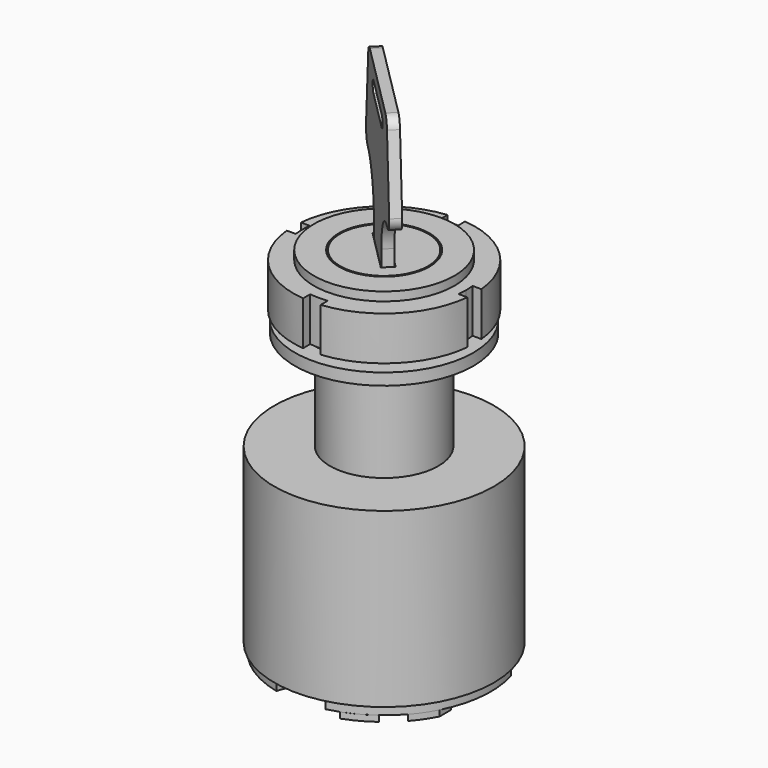
from build123d import *

# Parameters (mm, degrees)
F3_R      = 12
F4_DEPTH  = 7.5
F6_DEPTH  = 0.5
F7_R      = 7.75
F7_R_2    = 7.5
F8_DEPTH  = 0.5
F11_DEPTH = 0.875
F13_DEPTH = 1.5
F16_DEPTH = 1
F17_DEPTH = 1
F18_DEPTH = 1


# Not quite as in the source:
# - a feature names something its author has since deleted; it is built from what else it names


with BuildPart() as f1:
    # F0 (on Front) → F1 (revolve)
    with BuildSketch(Plane.XZ):
        Polygon((0, 59), (0, 0), (18.75, 0), (18.75, 29.5), (9.25, 29.5), (9.25, 44.5), (15.25, 46.5), (15.25, 48.5), (12, 48.5), (12, 59), align=None)
    revolve(axis=Axis((0, 0, 29.5), (0, 0, -1)))

    # F5 (on face) → F6 (cut)
    with BuildSketch(Plane.XY.offset(57.5)):
        with BuildLine():
            ThreePointArc((14.6735305908, 1.5), (14.7308702427, 0.7509739627), (14.75, 0))
            ThreePointArc((14.75, 0), (14.7308702427, -0.7509739627), (14.6735305908, -1.5))
            Line((14.6735305908, -1.5), (15.4272486205, -1.5))
            ThreePointArc((15.4272486205, -1.5), (15.4818014717, -0.750881609), (15.5, 0))
            ThreePointArc((15.5, 0), (15.4818014717, 0.750881609), (15.4272486205, 1.5))
            Line((15.4272486205, 1.5), (14.6735305908, 1.5))
        make_face()
        with BuildLine():
            ThreePointArc((-1.5, 14.6735305908), (0, 14.75), (1.5, 14.6735305908))
            Line((1.5, 14.6735305908), (1.5, 15.4272486205))
            ThreePointArc((1.5, 15.4272486205), (0, 15.5), (-1.5, 15.4272486205))
            Line((-1.5, 15.4272486205), (-1.5, 14.6735305908))
        make_face()
        with BuildLine():
            Line((1.5, -15.4272486205), (1.5, -14.6735305908))
            ThreePointArc((1.5, -14.6735305908), (0, -14.75), (-1.5, -14.6735305908))
            Line((-1.5, -14.6735305908), (-1.5, -15.4272486205))
            ThreePointArc((-1.5, -15.4272486205), (0, -15.5), (1.5, -15.4272486205))
        make_face()
        with BuildLine():
            ThreePointArc((-14.6735305908, -1.5), (-14.75, 0), (-14.6735305908, 1.5))
            Line((-14.6735305908, 1.5), (-15.4272486205, 1.5))
            ThreePointArc((-15.4272486205, 1.5), (-15.5, 0), (-15.4272486205, -1.5))
            Line((-15.4272486205, -1.5), (-14.6735305908, -1.5))
        make_face()
    extrude(amount=-F6_DEPTH, mode=Mode.SUBTRACT)

    # F7 (on face) → F8 (cut)
    with BuildSketch(Plane.XY.offset(59)):
        Circle(F7_R)
        Circle(F7_R_2, mode=Mode.SUBTRACT)
        Polygon((-2.8284271247, 4.2426406871), (-4.2426406871, 2.8284271247), (2.8284271247, -4.2426406871), (4.2426406871, -2.8284271247), (0, 1.4142135624), align=None)
    extrude(amount=-F8_DEPTH, mode=Mode.SUBTRACT)


with BuildPart() as f4:
    # F3 (on offset) → F4 (new body)
    with BuildSketch(Plane.XY.offset(50)):
        with BuildLine():
            Line((-1.5, 13.9194109071), (-1.5, 15.4272486205))
            ThreePointArc((-1.5, 15.4272486205), (-10.9601551084, 10.9601551084), (-15.4272486205, 1.5))
            Line((-15.4272486205, 1.5), (-13.9194109071, 1.5))
            ThreePointArc((-13.9194109071, 1.5), (-9.8994949366, 9.8994949366), (-1.5, 13.9194109071))
        make_face()
        with BuildLine():
            ThreePointArc((-1.5, -13.9194109071), (-9.8994949366, -9.8994949366), (-13.9194109071, -1.5))
            Line((-13.9194109071, -1.5), (-15.4272486205, -1.5))
            ThreePointArc((-15.4272486205, -1.5), (-10.9601551084, -10.9601551084), (-1.5, -15.4272486205))
            Line((-1.5, -15.4272486205), (-1.5, -13.9194109071))
        make_face()
        with BuildLine():
            ThreePointArc((13.9194109071, -1.5), (9.8994949366, -9.8994949366), (1.5, -13.9194109071))
            Line((1.5, -13.9194109071), (1.5, -15.4272486205))
            ThreePointArc((1.5, -15.4272486205), (10.9601551084, -10.9601551084), (15.4272486205, -1.5))
            Line((15.4272486205, -1.5), (13.9194109071, -1.5))
        make_face()
        with BuildLine():
            ThreePointArc((0, 14), (-0.7510816537, 13.979838209), (-1.5, 13.9194109071))
            ThreePointArc((-1.5, 13.9194109071), (-9.8994949366, 9.8994949366), (-13.9194109071, 1.5))
            ThreePointArc((-13.9194109071, 1.5), (-14, 0), (-13.9194109071, -1.5))
            ThreePointArc((-13.9194109071, -1.5), (-9.8994949366, -9.8994949366), (-1.5, -13.9194109071))
            ThreePointArc((-1.5, -13.9194109071), (0, -14), (1.5, -13.9194109071))
            ThreePointArc((1.5, -13.9194109071), (9.8994949366, -9.8994949366), (13.9194109071, -1.5))
            ThreePointArc((13.9194109071, -1.5), (13.979838209, -0.7510816537), (14, 0))
            ThreePointArc((14, 0), (13.979838209, 0.7510816537), (13.9194109071, 1.5))
            ThreePointArc((13.9194109071, 1.5), (9.8994949366, 9.8994949366), (1.5, 13.9194109071))
            ThreePointArc((1.5, 13.9194109071), (0.7510816537, 13.979838209), (0, 14))
        make_face()
        Circle(F3_R, mode=Mode.SUBTRACT)
        with BuildLine():
            Line((1.5, 15.4272486205), (1.5, 13.9194109071))
            ThreePointArc((1.5, 13.9194109071), (9.8994949366, 9.8994949366), (13.9194109071, 1.5))
            Line((13.9194109071, 1.5), (15.4272486205, 1.5))
            ThreePointArc((15.4272486205, 1.5), (10.9601551084, 10.9601551084), (1.5, 15.4272486205))
        make_face()
    extrude(amount=F4_DEPTH)


with BuildPart() as f11:
    # F10 (on offset) → F11 (new body, symmetric)
    with BuildSketch(Plane(origin=(0, 0, 0), x_dir=(0.7071067812, -0.7071067812, 0), z_dir=(-0.7071067812, -0.7071067812, 0))):
        with BuildLine():
            Line((-4.5, 58.5), (0, 58.5))
            Line((0, 58.5), (4.5, 58.5))
            Line((4.5, 58.5), (4.5, 61.5))
            ThreePointArc((4.5, 61.5), (6.5502525317, 66.4497474683), (11.5, 68.5))
            Line((11.5, 68.5), (12.0152075807, 68.5))
            ThreePointArc((12.0152075807, 68.5), (13.5732171306, 69.2459640187), (13.9690076155, 70.9273937576))
            Line((13.9690076155, 70.9273937576), (11.3440076155, 82.9273937576))
            ThreePointArc((11.3440076155, 82.9273937576), (10.644243562, 84.0580095499), (9.3902075807, 84.5))
            Line((9.3902075807, 84.5), (0, 84.5))
            Line((0, 84.5), (-9.3902075807, 84.5))
            ThreePointArc((-9.3902075807, 84.5), (-10.644243562, 84.0580095499), (-11.3440076155, 82.9273937576))
            Line((-11.3440076155, 82.9273937576), (-13.9690076155, 70.9273937576))
            ThreePointArc((-13.9690076155, 70.9273937576), (-13.5732171306, 69.2459640187), (-12.0152075807, 68.5))
            Line((-12.0152075807, 68.5), (-11.5, 68.5))
            ThreePointArc((-11.5, 68.5), (-6.5502525317, 66.4497474683), (-4.5, 61.5))
            Line((-4.5, 61.5), (-4.5, 58.5))
        make_face()
        with BuildLine():
            Line((-5, 82), (0, 82))
            Line((0, 82), (5, 82))
            ThreePointArc((5, 82), (6, 81), (5, 80))
            Line((5, 80), (0, 80))
            Line((0, 80), (-5, 80))
            ThreePointArc((-5, 80), (-6, 81), (-5, 82))
        make_face(mode=Mode.SUBTRACT)
    extrude(amount=F11_DEPTH, both=True)


with BuildPart() as f13:
    # F12 (on face) → F13 (new body)
    with BuildSketch(Plane(origin=(0, 0, 0), x_dir=(1, 0, 0), z_dir=(0, 0, -1))):
        with BuildLine():
            ThreePointArc((4.1808768461, 17.7646494139), (0, 14.2780423647), (-4.1808768461, 17.7646494139))
            ThreePointArc((-4.1808768461, 17.7646494139), (-15.8049636191, 9.125), (-17.4750761048, -5.2615791481))
            ThreePointArc((-17.4750761048, -5.2615791481), (-12.3651474041, -7.1390211823), (-13.2941992587, -12.5030702658))
            ThreePointArc((-13.2941992587, -12.5030702658), (0, -18.25), (13.2941992587, -12.5030702658))
            ThreePointArc((13.2941992587, -12.5030702658), (12.3651474041, -7.1390211823), (17.4750761048, -5.2615791481))
            ThreePointArc((17.4750761048, -5.2615791481), (15.8049636191, 9.125), (4.1808768461, 17.7646494139))
        make_face()
    extrude(amount=F13_DEPTH)

    # F15 (on face) → F18 (join)
    with BuildSketch(Plane(origin=(0, 0, -1.5), x_dir=(1, 0, 0), z_dir=(0, 0, -1))):
        with BuildLine():
            Line((16.1942188134, 6.1666581865), (16.1942188134, 8.4148545455))
            ThreePointArc((16.1942188134, 8.4148545455), (15.0551666883, 10.315253559), (13.6942188134, 12.0636176618))
            Line((13.6942188134, 12.0636176618), (13.6942188134, 8.6666581865))
            ThreePointArc((13.6942188134, 8.6666581865), (13.547772204, 8.3131047959), (13.1942188134, 8.1666581865))
            Line((13.1942188134, 8.1666581865), (6.6942188134, 8.1666581865))
            ThreePointArc((6.6942188134, 8.1666581865), (6.3406654228, 8.0202115771), (6.1942188134, 7.6666581865))
            Line((6.1942188134, 7.6666581865), (6.1942188134, 6.1666581865))
            ThreePointArc((6.1942188134, 6.1666581865), (6.3406654228, 5.8131047959), (6.6942188134, 5.6666581865))
            Line((6.6942188134, 5.6666581865), (15.6942188134, 5.6666581865))
            ThreePointArc((15.6942188134, 5.6666581865), (16.047772204, 5.8131047959), (16.1942188134, 6.1666581865))
        make_face()
    extrude(amount=F18_DEPTH)


with BuildPart() as f16:
    # F15 (on face) → F16 (new body)
    with BuildSketch(Plane(origin=(0, 0, -1.5), x_dir=(1, 0, 0), z_dir=(0, 0, -1))):
        with BuildLine():
            Line((-5, -16.25), (-5, -17.5517093185))
            ThreePointArc((-5, -17.5517093185), (0, -18.25), (5, -17.5517093185))
            Line((5, -17.5517093185), (5, -12.75))
            ThreePointArc((5, -12.75), (5.1464466094, -12.3964466094), (5.5, -12.25))
            Line((5.5, -12.25), (10.5, -12.25))
            ThreePointArc((10.5, -12.25), (10.8535533906, -12.1035533906), (11, -11.75))
            Line((11, -11.75), (11, -2.75))
            ThreePointArc((11, -2.75), (10.8535533906, -2.3964466094), (10.5, -2.25))
            Line((10.5, -2.25), (9, -2.25))
            ThreePointArc((9, -2.25), (8.6464466094, -2.3964466094), (8.5, -2.75))
            Line((8.5, -2.75), (8.5, -9.25))
            ThreePointArc((8.5, -9.25), (8.3535533906, -9.6035533906), (8, -9.75))
            Line((8, -9.75), (3, -9.75))
            ThreePointArc((3, -9.75), (2.6464466094, -9.6035533906), (2.5, -9.25))
            Line((2.5, -9.25), (2.5, -2.75))
            ThreePointArc((2.5, -2.75), (2.3535533906, -2.3964466094), (2, -2.25))
            Line((2, -2.25), (0.5, -2.25))
            ThreePointArc((0.5, -2.25), (0.1464466094, -2.3964466094), (0, -2.75))
            Line((0, -2.75), (0, -3.0306600966))
            Line((0, -3.0306600966), (-4.25, -3.0306600966))
            Line((-4.25, -3.0306600966), (-4.25, 5.5))
            ThreePointArc((-4.25, 5.5), (-4.3964466094, 5.8535533906), (-4.75, 6))
            Line((-4.75, 6), (-6.25, 6))
            ThreePointArc((-6.25, 6), (-6.6035533906, 5.8535533906), (-6.75, 5.5))
            Line((-6.75, 5.5), (-6.75, -1))
            ThreePointArc((-6.75, -1), (-6.8964466094, -1.3535533906), (-7.25, -1.5))
            Line((-7.25, -1.5), (-12.25, -1.5))
            ThreePointArc((-12.25, -1.5), (-12.6035533906, -1.3535533906), (-12.75, -1))
            Line((-12.75, -1), (-12.75, 5.5))
            ThreePointArc((-12.75, 5.5), (-12.8964466094, 5.8535533906), (-13.25, 6))
            Line((-13.25, 6), (-14.75, 6))
            ThreePointArc((-14.75, 6), (-15.1035533906, 5.8535533906), (-15.25, 5.5))
            Line((-15.25, 5.5), (-15.25, -3.5))
            ThreePointArc((-15.25, -3.5), (-15.1035533906, -3.8535533906), (-14.75, -4))
            Line((-14.75, -4), (-4.75, -4))
            ThreePointArc((-4.75, -4), (-4.3964466094, -3.8535533906), (-4.25, -3.5))
            Line((-4.25, -3.5), (-4.25, -3.1480044127))
            Line((-4.25, -3.1480044127), (0, -3.1480044127))
            Line((0, -3.1480044127), (0, -6.75))
            ThreePointArc((0, -6.75), (-0.1464466094, -7.1035533906), (-0.5, -7.25))
            Line((-0.5, -7.25), (-4.5, -7.25))
            ThreePointArc((-4.5, -7.25), (-4.8535533906, -7.3964466094), (-5, -7.75))
            Line((-5, -7.75), (-5, -9.25))
            ThreePointArc((-5, -9.25), (-4.8535533906, -9.6035533906), (-4.5, -9.75))
            Line((-4.5, -9.75), (2, -9.75))
            ThreePointArc((2, -9.75), (2.3535533906, -9.8964466094), (2.5, -10.25))
            Line((2.5, -10.25), (2.5, -15.25))
            ThreePointArc((2.5, -15.25), (2.3535533906, -15.6035533906), (2, -15.75))
            Line((2, -15.75), (0, -15.75))
            Line((0, -15.75), (-4.5, -15.75))
            ThreePointArc((-4.5, -15.75), (-4.8535533906, -15.8964466094), (-5, -16.25))
        make_face()
    extrude(amount=F16_DEPTH)


with BuildPart() as f17:
    # F15 (on face) → F17 (new body)
    with BuildSketch(Plane(origin=(0, 0, -1.5), x_dir=(1, 0, 0), z_dir=(0, 0, -1))):
        with BuildLine():
            ThreePointArc((10.8605542051, 14.6666581865), (8.6185161529, 16.0867547791), (6.1942188134, 17.1666581865))
            Line((6.1942188134, 17.1666581865), (6.1942188134, 15.1666581865))
            ThreePointArc((6.1942188134, 15.1666581865), (6.3406654228, 14.8131047959), (6.6942188134, 14.6666581865))
            Line((6.6942188134, 14.6666581865), (10.8605542051, 14.6666581865))
        make_face()
    extrude(amount=F17_DEPTH)


solid = Compound([f1.part, f4.part, f11.part, f13.part, f16.part, f17.part])
